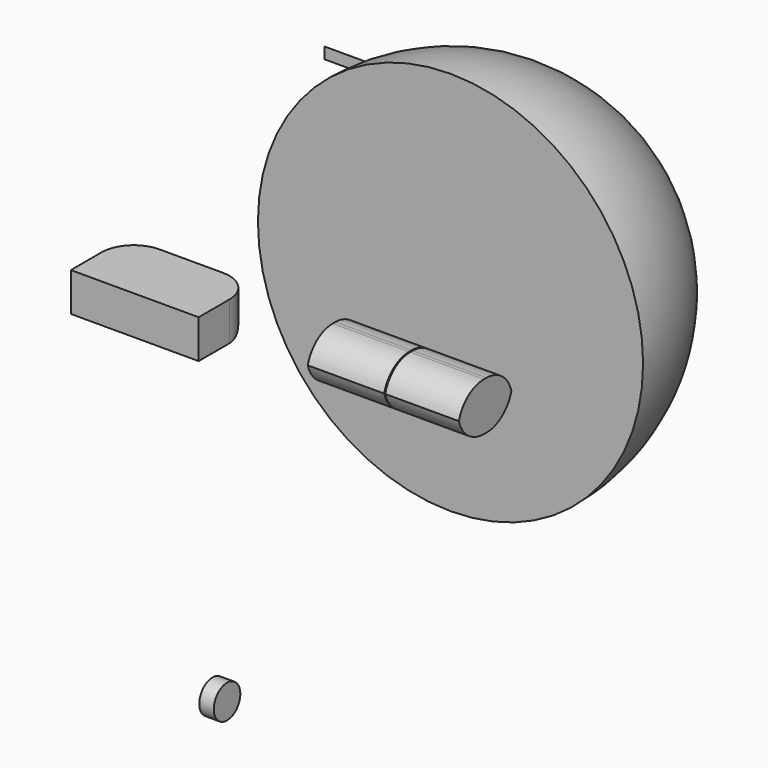
from build123d import *

# Parameters (mm, degrees)
F1_ANGLE      = 180
F2_W          = 11.6210272536
F2_H          = 10.6681920588
F3_DEPTH      = 7.62
F2_W_2        = 12.0515259914
F4_T1_DEPTH   = 37.0210272536
F4_2_T1_DEPTH = 37.4515259914
F5_R          = 2.6181603729
F6_DEPTH      = 2.286
F7_W          = 20.1528938487
F7_H          = 11.1292116344
F8_DEPTH      = 6.096
F9_R          = 5.08
F10_W         = 26.281952858
F10_H         = 1.7353892326
F11_DEPTH     = 2.54
F12_T1_DEPTH  = 48.2789981141


# Not quite as in the source:
# - a fillet or chamfer that OpenCascade refuses, or shapes differently, is made with other operations: its cross-section is extruded or revolved along the edge and cut away or added


with BuildPart() as f1:
    # F0 (on Front) → F1 (revolve)
    with BuildSketch(Plane.XZ):
        with BuildLine():
            Line((0, 0), (30.3797386587, 0))
            ThreePointArc((30.3797386587, 0), (0, 30.3797386587), (-30.3797386587, 0))
            Line((-30.3797386587, 0), (0, 0))
        make_face()
    revolve(axis=Axis((0, 0, 0), (-1, 0, 0)), revolution_arc=F1_ANGLE)


with BuildPart() as f3:
    # F2 (on Top) → F3 (new body)
    with BuildSketch(Plane.XY):
        with Locations((21.0152794607, -26.7067458481)):
            Rectangle(F2_W, F2_H)
    extrude(amount=F3_DEPTH)

    # F4: fillet of radius 5.08 on 4 edges, made by hand

    # F4_s2 → F4_t1 (cut)
    with BuildSketch(Plane.YZ.offset(2.5047658339)):
        with BuildLine():
            ThreePointArc((-21.3726498187, 5.08), (-22.8605473702, 1.4878975516), (-26.4526498187, 0))
            Line((-26.4526498187, 0), (-21.3726498187, 0))
            Line((-21.3726498187, 0), (-21.3726498187, 5.08))
        make_face()
        with BuildLine():
            ThreePointArc((-32.0408418775, 5.08), (-30.5529443259, 1.4878975516), (-26.9608418775, 0))
            Line((-26.9608418775, 0), (-32.0408418775, 0))
            Line((-32.0408418775, 0), (-32.0408418775, 5.08))
        make_face()
        with BuildLine():
            ThreePointArc((-32.0408418775, 2.54), (-30.5529443259, 6.1321024484), (-26.9608418775, 7.62))
            Line((-26.9608418775, 7.62), (-32.0408418775, 7.62))
            Line((-32.0408418775, 7.62), (-32.0408418775, 2.54))
        make_face()
        with BuildLine():
            ThreePointArc((-21.3726498187, 2.54), (-22.8605473702, 6.1321024484), (-26.4526498187, 7.62))
            Line((-26.4526498187, 7.62), (-21.3726498187, 7.62))
            Line((-21.3726498187, 7.62), (-21.3726498187, 2.54))
        make_face()
    extrude(amount=F4_T1_DEPTH, mode=Mode.SUBTRACT)


with BuildPart() as f3b:
    # F2 (on Top) → F3, piece 2 (new body)
    with BuildSketch(Plane.XY):
        with Locations((9.0137117077, -26.7067458481)):
            Rectangle(F2_W_2, F2_H)
    extrude(amount=F3_DEPTH)

    # F4#2: fillet of radius 5.08 on 4 edges, made by hand

    # F4_2_s2 → F4_2_t1 (cut)
    with BuildSketch(Plane.YZ.offset(-9.712051288)):
        with BuildLine():
            ThreePointArc((-21.3726498187, 5.08), (-22.8605473702, 1.4878975516), (-26.4526498187, 0))
            Line((-26.4526498187, 0), (-21.3726498187, 0))
            Line((-21.3726498187, 0), (-21.3726498187, 5.08))
        make_face()
        with BuildLine():
            ThreePointArc((-32.0408418775, 5.08), (-30.5529443259, 1.4878975516), (-26.9608418775, 0))
            Line((-26.9608418775, 0), (-32.0408418775, 0))
            Line((-32.0408418775, 0), (-32.0408418775, 5.08))
        make_face()
        with BuildLine():
            ThreePointArc((-32.0408418775, 2.54), (-30.5529443259, 6.1321024484), (-26.9608418775, 7.62))
            Line((-26.9608418775, 7.62), (-32.0408418775, 7.62))
            Line((-32.0408418775, 7.62), (-32.0408418775, 2.54))
        make_face()
        with BuildLine():
            ThreePointArc((-21.3726498187, 2.54), (-22.8605473702, 6.1321024484), (-26.4526498187, 7.62))
            Line((-26.4526498187, 7.62), (-21.3726498187, 7.62))
            Line((-21.3726498187, 7.62), (-21.3726498187, 2.54))
        make_face()
    extrude(amount=F4_2_T1_DEPTH, mode=Mode.SUBTRACT)


with BuildPart() as f6:
    # F5 (on Right) → F6 (new body)
    with BuildSketch(Plane.YZ):
        with Locations((-46.923160553, -36.9971059263)):
            Circle(F5_R)
    extrude(amount=F6_DEPTH)


with BuildPart() as f8:
    # F7 (on Top) → F8 (new body)
    with BuildSketch(Plane.XY):
        with Locations((-22.8599994443, -28.1238164753)):
            Rectangle(F7_W, F7_H)
    extrude(amount=F8_DEPTH)

    # F9
    f9_edges = [f8.edges().sort_by_distance(p)[0] for p in [
        (-12.783553, -22.559211, 3.048),
        (-32.936446, -22.559211, 3.048),
        (-22.859999, -22.559211, 0),
    ]]
    fillet(f9_edges, radius=F9_R)


with BuildPart() as f11:
    # F10 (on Top) → F11 (new body)
    with BuildSketch(Plane.XY):
        with Locations((-37.8428399563, 39.738882333)):
            Rectangle(F10_W, F10_H)
    extrude(amount=F11_DEPTH)

    # F12: fillet of radius 5.08 on 1 edges, made by hand

    # F12_s2 → F12_t1 (cut)
    with BuildSketch(Plane.YZ.offset(-61.9823390133)):
        with BuildLine():
            ThreePointArc((40.6065769494, 0), (38.7471678981, 1.8594090512), (36.2071678981, 2.54))
            Line((36.2071678981, 2.54), (40.6065769494, 2.54))
            Line((40.6065769494, 2.54), (40.6065769494, 0))
        make_face()
    extrude(amount=F12_T1_DEPTH, mode=Mode.SUBTRACT)


solid = Compound([f1.part, f3.part, f3b.part, f6.part, f8.part, f11.part])
